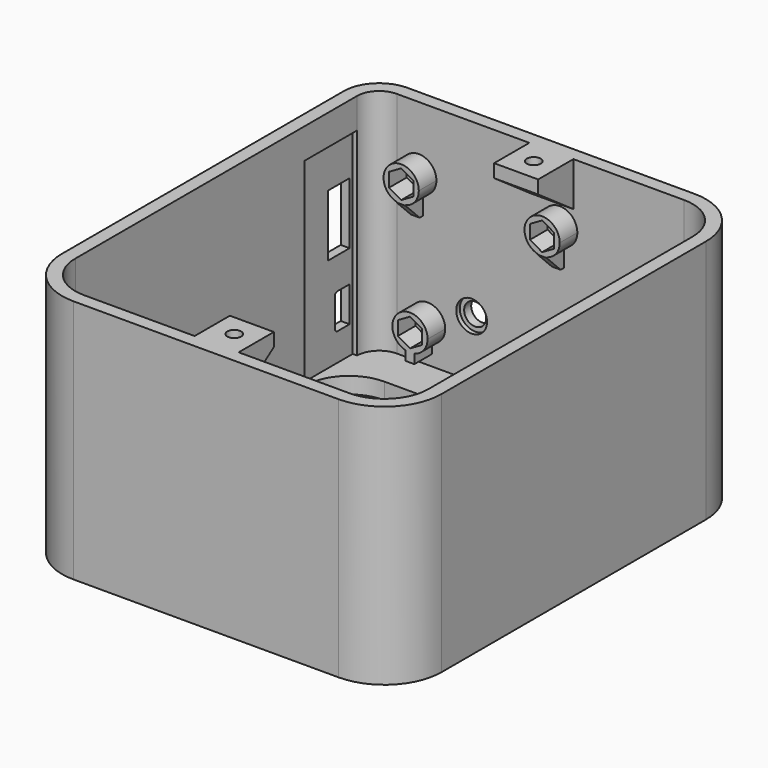
from build123d import *

# Parameters (mm, degrees)
F1_DEPTH  = 3.7
F2_DEPTH  = 55.6
F5_DEPTH  = 5
F7_D      = 3.15
F7_DEPTH  = 10
F7_TIP    = 0.946355475
F9_R      = 3
F10_DEPTH = 10
F12_DEPTH = 5
F11_R     = 2.5
F13_DEPTH = 25
F11_R_2   = 3.5
F14_DEPTH = 1
F15_SIZE  = 4
F16_W     = 4.2
F16_H     = 8
F16_W_2   = 6.1
F16_H_2   = 14
F17_DEPTH = 1
F18_DEPTH = 3
F19_R     = 0.8


with BuildPart() as f1:
    # F0 (on Top) → F1 (new body)
    with BuildSketch(Plane.XY):
        with BuildLine():
            ThreePointArc((43.1, 37.5), (39.2923881554, 46.6923881554), (30.1, 50.5))
            Line((30.1, 50.5), (-35.1, 50.5))
            ThreePointArc((-35.1, 50.5), (-40.7568542495, 48.1568542495), (-43.1, 42.5))
            Line((-43.1, 42.5), (-43.1, -37.5))
            ThreePointArc((-43.1, -37.5), (-39.2923881554, -46.6923881554), (-30.1, -50.5))
            Line((-30.1, -50.5), (30.1, -50.5))
            ThreePointArc((30.1, -50.5), (39.2923881554, -46.6923881554), (43.1, -37.5))
            Line((43.1, -37.5), (43.1, 37.5))
        make_face()
        with BuildLine():
            Line((40.1, 37.5), (40.1, 27.7))
            Line((40.1, 27.7), (40.1, -37.5))
            ThreePointArc((40.1, -37.5), (37.1710678119, -44.5710678119), (30.1, -47.5))
            Line((30.1, -47.5), (-30.1, -47.5))
            ThreePointArc((-30.1, -47.5), (-37.1710678119, -44.5710678119), (-40.1, -37.5))
            Line((-40.1, -37.5), (-40.1, 27.7))
            Line((-40.1, 27.7), (-40.1, 42.5))
            ThreePointArc((-40.1, 42.5), (-38.6355339059, 46.0355339059), (-35.1, 47.5))
            Line((-35.1, 47.5), (30.1, 47.5))
            ThreePointArc((30.1, 47.5), (37.1710678119, 44.5710678119), (40.1, 37.5))
        make_face(mode=Mode.SUBTRACT)
        with BuildLine():
            Line((-30.1, 37.7), (30.1, 37.7))
            ThreePointArc((30.1, 37.7), (37.1710678119, 34.7710678119), (40.1, 27.7))
            Line((40.1, 27.7), (40.1, 37.5))
            ThreePointArc((40.1, 37.5), (37.1710678119, 44.5710678119), (30.1, 47.5))
            Line((30.1, 47.5), (-35.1, 47.5))
            ThreePointArc((-35.1, 47.5), (-38.6355339059, 46.0355339059), (-40.1, 42.5))
            Line((-40.1, 42.5), (-40.1, 27.7))
            ThreePointArc((-40.1, 27.7), (-37.1710678119, 34.7710678119), (-30.1, 37.7))
        make_face()
    extrude(amount=F1_DEPTH)

    # F0 (on Top) → F2 (join)
    with BuildSketch(Plane.XY):
        with BuildLine():
            ThreePointArc((43.1, 37.5), (39.2923881554, 46.6923881554), (30.1, 50.5))
            Line((30.1, 50.5), (-35.1, 50.5))
            ThreePointArc((-35.1, 50.5), (-40.7568542495, 48.1568542495), (-43.1, 42.5))
            Line((-43.1, 42.5), (-43.1, -37.5))
            ThreePointArc((-43.1, -37.5), (-39.2923881554, -46.6923881554), (-30.1, -50.5))
            Line((-30.1, -50.5), (30.1, -50.5))
            ThreePointArc((30.1, -50.5), (39.2923881554, -46.6923881554), (43.1, -37.5))
            Line((43.1, -37.5), (43.1, 37.5))
        make_face()
        with BuildLine():
            Line((40.1, 37.5), (40.1, 27.7))
            Line((40.1, 27.7), (40.1, -37.5))
            ThreePointArc((40.1, -37.5), (37.1710678119, -44.5710678119), (30.1, -47.5))
            Line((30.1, -47.5), (-30.1, -47.5))
            ThreePointArc((-30.1, -47.5), (-37.1710678119, -44.5710678119), (-40.1, -37.5))
            Line((-40.1, -37.5), (-40.1, 27.7))
            Line((-40.1, 27.7), (-40.1, 42.5))
            ThreePointArc((-40.1, 42.5), (-38.6355339059, 46.0355339059), (-35.1, 47.5))
            Line((-35.1, 47.5), (30.1, 47.5))
            ThreePointArc((30.1, 47.5), (37.1710678119, 44.5710678119), (40.1, 37.5))
        make_face(mode=Mode.SUBTRACT)
    extrude(amount=F2_DEPTH)

    # F4 (on offset) → F5 (join, symmetric)
    with BuildSketch(Plane(origin=(0, 0, 0), x_dir=(0, -1, 0), z_dir=(-1, 0, 0))):
        Polygon((47.5, 45.6), (47.5, 55.6), (37.5, 55.6), (37.5, 52.6), align=None)
        Polygon((-37.5, 52.6), (-37.5, 55.6), (-47.5, 55.6), (-47.5, 45.6), align=None)
    extrude(amount=F5_DEPTH, both=True)

    # F7
    with Locations(Plane.XY.offset(55.6)):
        with Locations((0, 42.5), (0, -42.5)):
            Hole(F7_D / 2, depth=F7_DEPTH)
            with Locations((0, 0, -(F7_DEPTH + F7_TIP / 2))):  # 118° drill point
                Cone(0, F7_D / 2, F7_TIP, mode=Mode.SUBTRACT)

    # F9 (on offset) → F10 (cut)
    with BuildSketch(Plane.XY.offset(52.6)):
        with Locations((0, 42.5)):
            Circle(F9_R)
        with Locations((0, -42.5)):
            Circle(F9_R)
    extrude(amount=-F10_DEPTH, mode=Mode.SUBTRACT)

    # F11 (on face) → F12 (join)
    with BuildSketch(Plane.XZ.offset(-47.5)):
        with BuildLine():
            ThreePointArc((-29.1, 37.3270166538), (-26.9377223398, 38.7505102572), (-26.1, 41.2))
            ThreePointArc((-26.1, 41.2), (-32.5494897428, 44.3622776602), (-31.1, 37.3270166538))
            ThreePointArc((-31.1, 37.3270166538), (-30.1, 37.2), (-29.1, 37.3270166538))
        make_face()
        Polygon((-30.1, 44.3754264805), (-27.35, 42.7877132403), (-27.35, 39.6122867597), (-30.1, 38.0245735195), (-32.85, 39.6122867597), (-32.85, 42.7877132403), align=None, mode=Mode.SUBTRACT)
        with BuildLine():
            ThreePointArc((-29.1, 37.3270166538), (-30.1, 37.2), (-31.1, 37.3270166538))
            Line((-31.1, 37.3270166538), (-31.1, 33.2))
            Line((-31.1, 33.2), (-29.1, 33.2))
            Line((-29.1, 33.2), (-29.1, 37.3270166538))
        make_face()
        with BuildLine():
            ThreePointArc((2.9, 37.3270166538), (5.0622776602, 38.7505102572), (5.9, 41.2))
            ThreePointArc((5.9, 41.2), (-0.5494897428, 44.3622776602), (0.9, 37.3270166538))
            ThreePointArc((0.9, 37.3270166538), (1.9, 37.2), (2.9, 37.3270166538))
        make_face()
        Polygon((1.9, 44.3754264805), (4.65, 42.7877132403), (4.65, 39.6122867597), (1.9, 38.0245735195), (-0.85, 39.6122867597), (-0.85, 42.7877132403), align=None, mode=Mode.SUBTRACT)
        with BuildLine():
            ThreePointArc((2.9, 37.3270166538), (1.9, 37.2), (0.9, 37.3270166538))
            Line((0.9, 37.3270166538), (0.9, 33.2))
            Line((0.9, 33.2), (2.9, 33.2))
            Line((2.9, 33.2), (2.9, 37.3270166538))
        make_face()
        with BuildLine():
            ThreePointArc((-27.1, 8.3270166538), (-24.9377223398, 9.7505102572), (-24.1, 12.2))
            ThreePointArc((-24.1, 12.2), (-30.5494897428, 15.3622776602), (-29.1, 8.3270166538))
            ThreePointArc((-29.1, 8.3270166538), (-28.1, 8.2), (-27.1, 8.3270166538))
        make_face()
        Polygon((-28.1, 15.3754264805), (-25.35, 13.7877132403), (-25.35, 10.6122867597), (-28.1, 9.0245735195), (-30.85, 10.6122867597), (-30.85, 13.7877132403), align=None, mode=Mode.SUBTRACT)
        with BuildLine():
            ThreePointArc((-27.1, 8.3270166538), (-28.1, 8.2), (-29.1, 8.3270166538))
            Line((-29.1, 8.3270166538), (-29.1, 6.2))
            Line((-29.1, 6.2), (-27.1, 6.2))
            Line((-27.1, 6.2), (-27.1, 8.3270166538))
        make_face()
        with BuildLine():
            ThreePointArc((5.9, 8.3270166538), (8.0622776602, 9.7505102572), (8.9, 12.2))
            ThreePointArc((8.9, 12.2), (2.4505102572, 15.3622776602), (3.9, 8.3270166538))
            ThreePointArc((3.9, 8.3270166538), (4.9, 8.2), (5.9, 8.3270166538))
        make_face()
        Polygon((4.9, 15.3754264805), (7.65, 13.7877132403), (7.65, 10.6122867597), (4.9, 9.0245735195), (2.15, 10.6122867597), (2.15, 13.7877132403), align=None, mode=Mode.SUBTRACT)
        with BuildLine():
            ThreePointArc((5.9, 8.3270166538), (4.9, 8.2), (3.9, 8.3270166538))
            Line((3.9, 8.3270166538), (3.9, 6.2))
            Line((3.9, 6.2), (5.9, 6.2))
            Line((5.9, 6.2), (5.9, 8.3270166538))
        make_face()
    extrude(amount=F12_DEPTH)

    # F11 (on face) → F13 (cut)
    with BuildSketch(Plane.XZ.offset(-47.5)):
        with Locations((-18.1, 16.7)):
            Circle(F11_R)
    extrude(amount=-F13_DEPTH, mode=Mode.SUBTRACT)

    # F11 (on face) → F14 (cut)
    with BuildSketch(Plane.XZ.offset(-47.5)):
        with Locations((-18.1, 16.7)):
            Circle(F11_R_2)
        with Locations((-18.1, 16.7)):
            Circle(F11_R, mode=Mode.SUBTRACT)
        with Locations((-18.1, 16.7)):
            Circle(F11_R)
    extrude(amount=-F14_DEPTH, mode=Mode.SUBTRACT)

    # F15
    f15_edges = [f1.edges().sort_by_distance(p)[0] for p in [
        (1.9, 42.5, 33.2),
        (-30.1, 42.5, 33.2),
    ]]
    chamfer(f15_edges, length=F15_SIZE)

    # F16 (on face) → F17 (cut)
    with BuildSketch(Plane.YZ.offset(-40.1)):
        Polygon((27.7, 3.7), (42.5, 3.7), (42.5, 48.7), (27.5, 48.7), (27.5, 3.7), align=None)
        with Locations((39.5, 14)):
            Rectangle(F16_W, F16_H, mode=Mode.SUBTRACT)
        with Locations((38.55, 32.2)):
            Rectangle(F16_W_2, F16_H_2, mode=Mode.SUBTRACT)
    extrude(amount=-F17_DEPTH, mode=Mode.SUBTRACT)

    # F16 (on face) → F18 (cut)
    with BuildSketch(Plane.YZ.offset(-40.1)):
        with Locations((38.55, 32.2)):
            Rectangle(F16_W_2, F16_H_2)
        with Locations((39.5, 14)):
            Rectangle(F16_W, F16_H)
    extrude(amount=-F18_DEPTH, mode=Mode.SUBTRACT)

    # F19
    f19_edges = [f1.edges().sort_by_distance(p)[0] for p in [
        (-42.1, 37.4, 18),
        (-42.1, 37.4, 10),
    ]]
    fillet(f19_edges, radius=F19_R)


solid = f1.part
